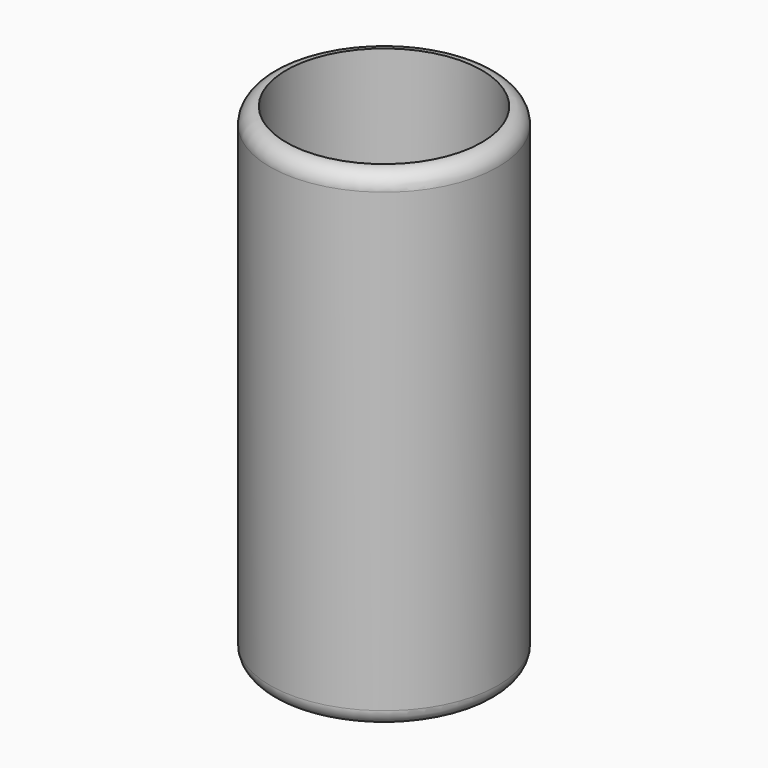
from build123d import *

# Parameters (mm, degrees)
F0_R     = 35
F0_R_2   = 30
F1_DEPTH = 150
F2_R     = 4.99999


# Not quite as in the source:
# - a fillet or chamfer is up to 0.001 mm smaller than in the source, because OpenCascade refuses the exact size


with BuildPart() as f1:
    # F0 (on Top) → F1 (new body)
    with BuildSketch(Plane.XY):
        Circle(F0_R)
        Circle(F0_R_2, mode=Mode.SUBTRACT)
    extrude(amount=F1_DEPTH)

    # F2 (radius 5 in the source; OpenCascade refuses exactly that, so slightly less here)
    f2_edges = [f1.edges().sort_by_distance(p)[0] for p in [
        (-35, 0, 150),
        (-35, 0, 0),
    ]]
    fillet(f2_edges, radius=F2_R)


solid = f1.part
